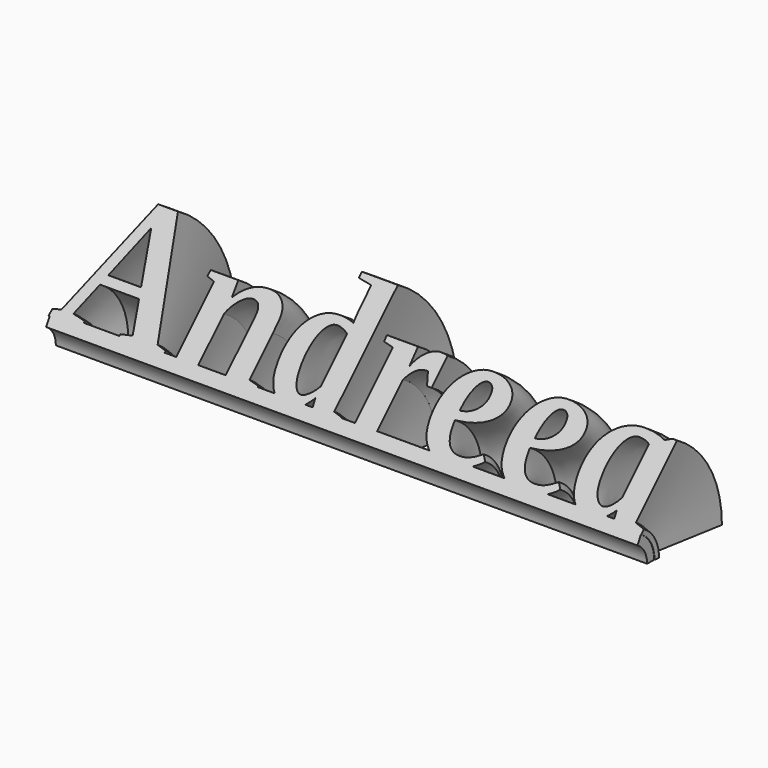
from build123d import *

# Parameters (mm, degrees)
F0_TEXT_SIZE = 41.2964533704
F1_W         = 144.3423703313
F1_H         = 3.2436503097
F3_ANGLE     = 60


# Not quite as in the source:
# - Text() gives the source's letters only with a copy of the font that has no kerning and outlines rounded to 1/6400 em; it was checked with that copy


with BuildPart() as f3:
    # F0 (on Top) + F1 (on Top) → F3 (revolve)
    with BuildSketch(Plane.XY):
        with Locations((-76.1581659317, -14.5288435742)):
            Text('Andreea', F0_TEXT_SIZE, font='Tinos', font_style=FontStyle.BOLDITALIC, text_align=(TextAlign.LEFT, TextAlign.BOTTOM))
    with BuildSketch(Plane.XY):
        with Locations((-5.8791153133, -15.0694516487)):
            Rectangle(F1_W, F1_H)
    revolve(axis=Axis((2.5003142655, -22.6379651576, 0), (1, 0, 0)), revolution_arc=F3_ANGLE)


solid = f3.part
